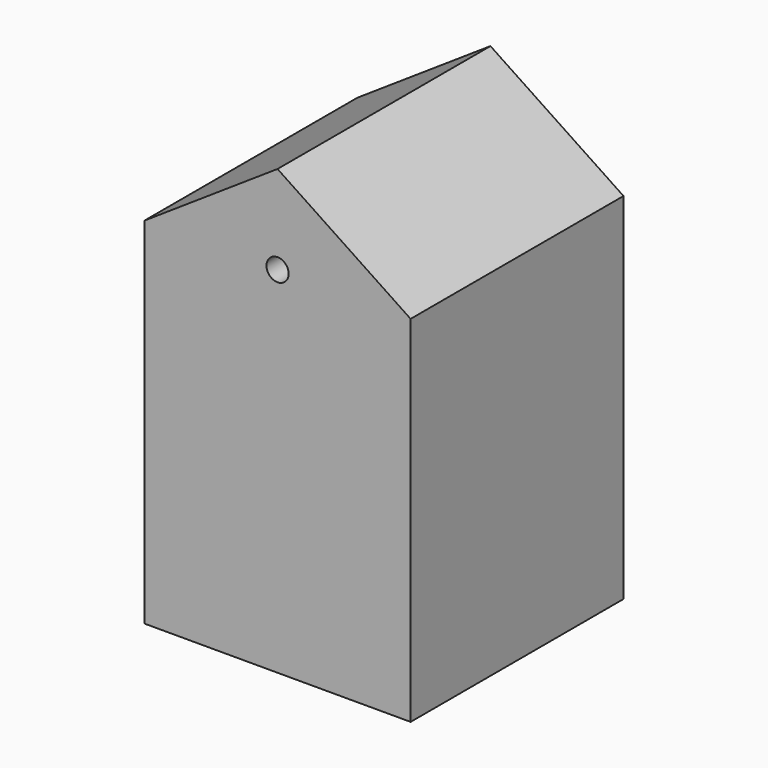
from build123d import *

# Parameters (mm, degrees)
F1_DEPTH = 38.1
F2_T     = -6.35
F5_R     = 3.2075388265
F6_DEPTH = 77.5145
F7_R     = 3.175
F8_DEPTH = 38.101


# Not quite as in the source:
# - a feature of the source that left no trace in its solid (it failed there, or was rolled back) is left out
# - the program builds the solid bodies; features that only make, move or delete a surface that nothing else refers to are left out


with BuildPart() as f1:
    # F0 (on Front) → F1 (new body, symmetric)
    with BuildSketch(Plane.XZ):
        Polygon((-38.1, 50.8), (-38.1, -50.8), (38.1, -50.8), (38.1, 50.8), (0, 76.2), align=None)
    extrude(amount=F1_DEPTH, both=True)

    # F2
    f2_openings = [f1.faces().sort_by_distance(p)[0] for p in [
        (0, 38.1, 6.585185),
    ]]
    offset(amount=F2_T, openings=f2_openings)

    # F5 (on face) → F6 (join)
    with BuildSketch(Plane.XY.offset(-44.45)):
        with Locations((0.0866505507, 6.0838097706)):
            Circle(F5_R)
    extrude(amount=F6_DEPTH)

    # F7 (on face) → F8 (cut, through all)
    with BuildSketch(Plane.XZ):
        with Locations((0, 50.8)):
            Circle(F7_R)
    extrude(amount=F8_DEPTH, mode=Mode.SUBTRACT)


solid = f1.part
